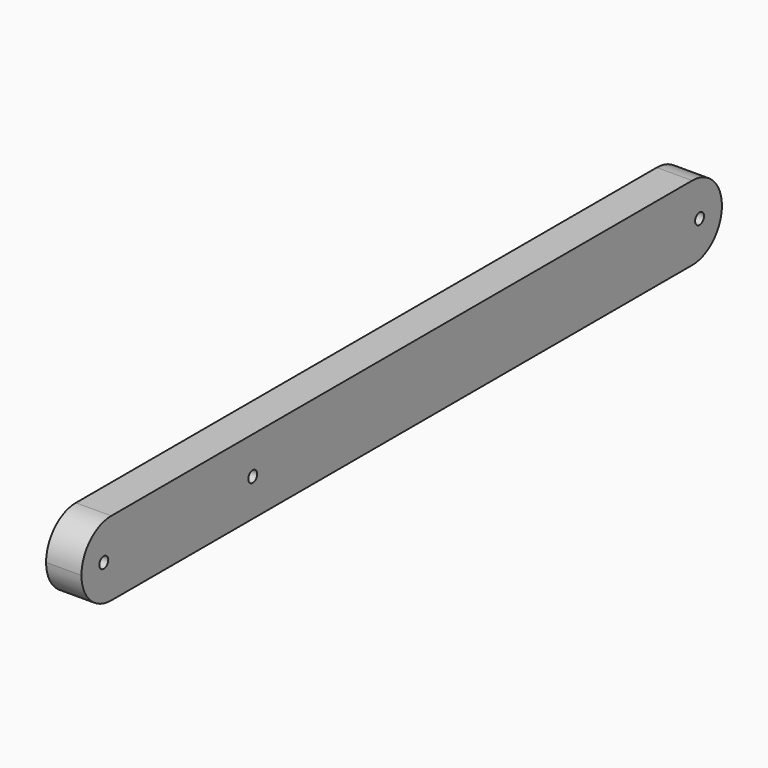
from build123d import *

# Parameters (mm, degrees)
F0_W     = 430
F0_H     = 40
F0_R     = 3
F1_DEPTH = 19
F2_R     = 19.99999
F3_R     = 3
F4_DEPTH = 19.001


# Not quite as in the source:
# - a fillet or chamfer is up to 0.001 mm smaller than in the source, because OpenCascade refuses the exact size


with BuildPart() as f1:
    # F0 (on Right) → F1 (new body)
    with BuildSketch(Plane.YZ):
        with Locations((-200, 0)):
            Rectangle(F0_W, F0_H)
        with Locations((-400, 0)):
            Circle(F0_R, mode=Mode.SUBTRACT)
        Circle(F0_R, mode=Mode.SUBTRACT)
    extrude(amount=F1_DEPTH)

    # F2 (radius 20 in the source; OpenCascade refuses exactly that, so slightly less here)
    f2_edges = [f1.edges().sort_by_distance(p)[0] for p in [
        (9.5, 15, 20),
        (9.5, 15, -20),
        (9.5, -415, 20),
        (9.5, -415, -20),
    ]]
    fillet(f2_edges, radius=F2_R)

    # F3 (on face) → F4 (cut, through all)
    with BuildSketch(Plane.YZ.offset(19)):
        with Locations((-300, 0)):
            Circle(F3_R)
    extrude(amount=-F4_DEPTH, mode=Mode.SUBTRACT)


solid = f1.part
